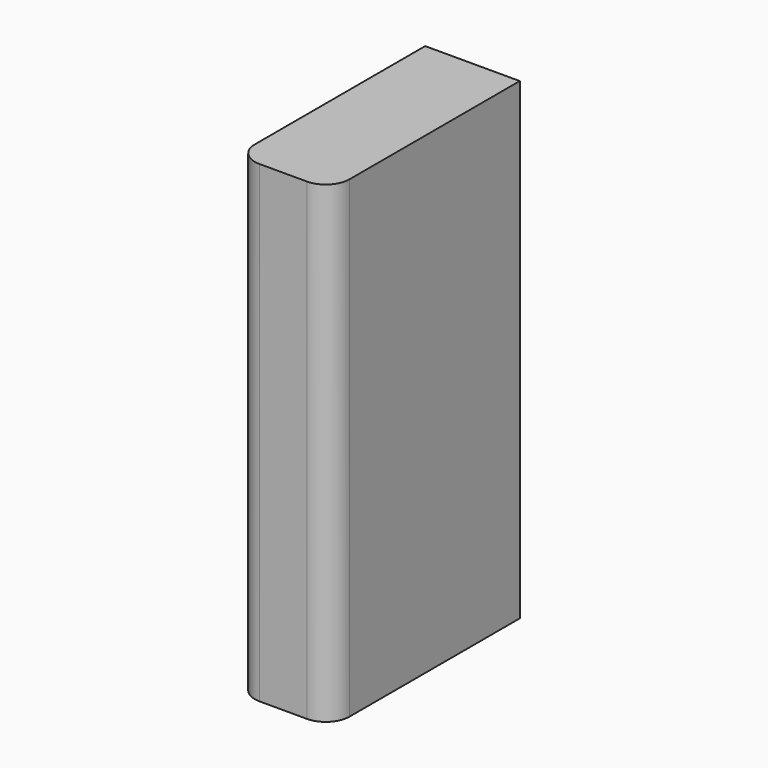
from build123d import *

# Parameters (mm, degrees)
F0_W     = 1000
F0_H     = 2000
F1_DEPTH = 400
F2_R     = 100


# Not quite as in the source:
# - a feature of the source that left no trace in its solid (it failed there, or was rolled back) is left out


with BuildPart() as f1:
    # F0 (on Right) → F1 (new body)
    with BuildSketch(Plane.YZ):
        with Locations((-500, 1000)):
            Rectangle(F0_W, F0_H)
    extrude(amount=F1_DEPTH)

    # F2
    f2_edges = [f1.edges().sort_by_distance(p)[0] for p in [
        (0, -1000, 1000),
        (400, -1000, 1000),
    ]]
    fillet(f2_edges, radius=F2_R)


solid = f1.part
